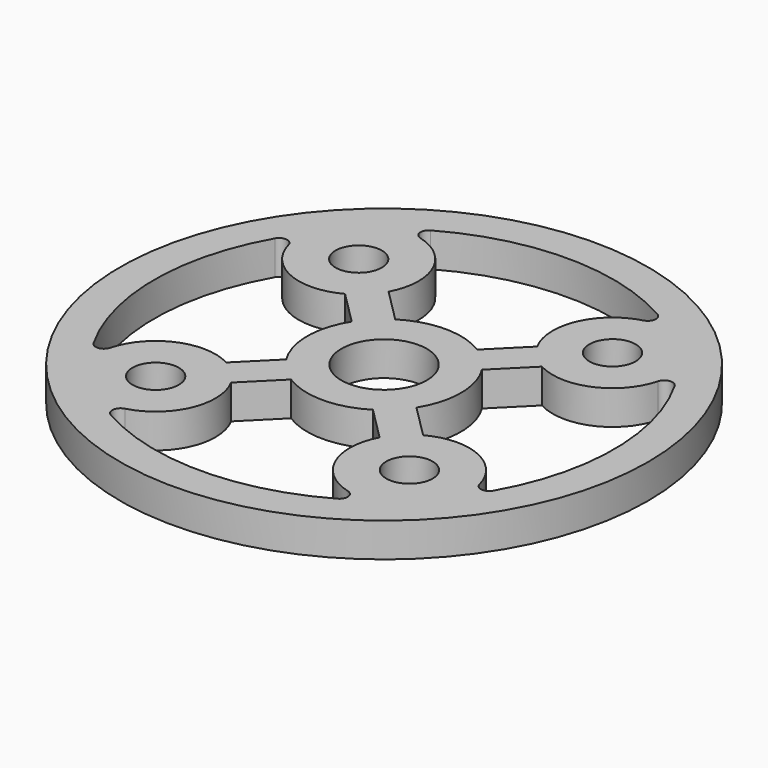
from build123d import *

# Parameters (mm, degrees)
F0_R            = 24.51608
F0_R_2          = 2.15265
F0_R_3          = 3.96875
F1_DEPTH        = 3.175
F3_DEPTH        = 3.175
F3_COPIES_COUNT = 4
F4_R            = 0.762


# Not quite as in the source:
# - a pattern or mirror of a feature is missing from the dataset's text; its kind, count and spacing are read off the source's solid


with BuildPart() as f1:
    # F0 (on Top) → F1 (new body)
    with BuildSketch(Plane.XY):
        Circle(F0_R)
        with Locations((-11.7865906, -11.7865906)):
            Circle(F0_R_2, mode=Mode.SUBTRACT)
        with Locations((11.7865906, -11.7865906)):
            Circle(F0_R_2, mode=Mode.SUBTRACT)
        with Locations((-11.7865906, 11.7865906)):
            Circle(F0_R_2, mode=Mode.SUBTRACT)
        Circle(F0_R_3, mode=Mode.SUBTRACT)
        with Locations((11.7865906, 11.7865906)):
            Circle(F0_R_2, mode=Mode.SUBTRACT)
    extrude(amount=F1_DEPTH)

    # F2 (on face) → F3 (cut, through all)
    with BuildSketch(Plane.XY.offset(3.175)):
        with BuildLine():
            ThreePointArc((-12.5005198818, 17.2967828873), (-7.207099086, 14.9330444032), (-6.8989717457, 9.144035776))
            Line((-6.8989717457, 9.144035776), (-3.8025572131, 6.0476212434))
            ThreePointArc((-3.8025572131, 6.0476212434), (0, 7.14375), (3.8025572131, 6.0476212434))
            Line((3.8025572131, 6.0476212434), (6.8989717457, 9.144035776))
            ThreePointArc((6.8989717457, 9.144035776), (7.207099086, 14.9330444032), (12.5005198818, 17.2967828873))
            ThreePointArc((12.5005198818, 17.2967828873), (0, 21.34108), (-12.5005198818, 17.2967828873))
        make_face()
    f3 = extrude(amount=-F3_DEPTH, mode=Mode.SUBTRACT)

    # F3_copies: F3 ×4 about axis
    f3_copies_axis = Axis((0, 0, 0), (0, 0, 1))
    for i in range(1, F3_COPIES_COUNT):
        add(f3.rotate(f3_copies_axis, i * 360 / F3_COPIES_COUNT), mode=Mode.SUBTRACT)

    # F4
    f4_edges = [f1.edges().sort_by_distance(p)[0] for p in [
        (-12.50052, 17.296783, 1.5875),
        (12.50052, 17.296783, 1.5875),
        (12.50052, -17.296783, 1.5875),
        (-12.50052, -17.296783, 1.5875),
        (17.296783, 12.50052, 1.5875),
        (17.296783, -12.50052, 1.5875),
        (-17.296783, -12.50052, 1.5875),
        (-17.296783, 12.50052, 1.5875),
    ]]
    fillet(f4_edges, radius=F4_R)


solid = f1.part
